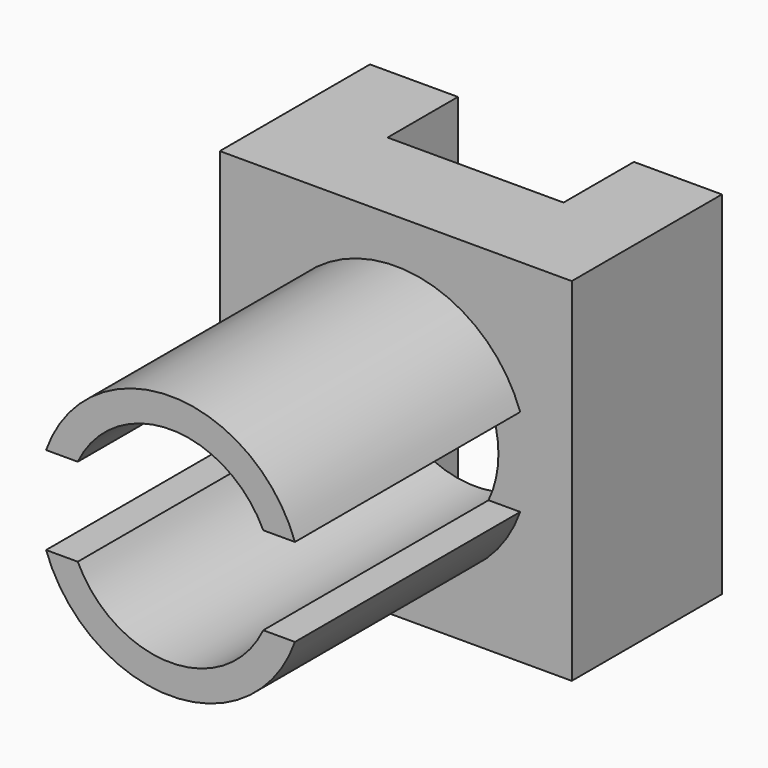
from build123d import *

# Parameters (mm, degrees)
F0_R     = 22.5
F0_R_2   = 17.5
F1_DEPTH = 48
F2_W     = 60
F2_H     = 60
F2_R     = 22.5
F2_R_2   = 17.5
F3_DEPTH = 32
F4_W     = 30
F4_H     = 15
F5_DEPTH = 60.001
F7_DEPTH = 48


with BuildPart() as f1:
    # F0 (on Front) → F1 (new body)
    with BuildSketch(Plane.XZ):
        Circle(F0_R)
        Circle(F0_R_2, mode=Mode.SUBTRACT)
    extrude(amount=F1_DEPTH)

    # F2 (on face) → F3 (join)
    with BuildSketch(Plane(origin=(0, 0, 0), x_dir=(-1, 0, 0), z_dir=(0, 1, 0))):
        Rectangle(F2_W, F2_H)
        Circle(F2_R, mode=Mode.SUBTRACT)
        Circle(F2_R)
        Circle(F2_R_2, mode=Mode.SUBTRACT)
    extrude(amount=F3_DEPTH)

    # F4 (on face) → F5 (cut, through all)
    with BuildSketch(Plane(origin=(0, 0, -30), x_dir=(1, 0, 0), z_dir=(0, 0, -1))):
        with Locations((0, -24.5)):
            Rectangle(F4_W, F4_H)
    extrude(amount=-F5_DEPTH, mode=Mode.SUBTRACT)

    # F6 (on face) → F7 (cut, through all)
    with BuildSketch(Plane.XZ.offset(48)):
        with BuildLine():
            ThreePointArc((-21.2132034356, 7.5), (-22.5, 0), (-21.2132034356, -7.5))
            Line((-21.2132034356, -7.5), (-15.8113883008, -7.5))
            ThreePointArc((-15.8113883008, -7.5), (-17.5, 0), (-15.8113883008, 7.5))
            Line((-15.8113883008, 7.5), (-21.2132034356, 7.5))
        make_face()
        with BuildLine():
            Line((15.8113883008, -7.5), (21.2132034356, -7.5))
            ThreePointArc((21.2132034356, -7.5), (22.1759675922, -3.8047945213), (22.5, 0))
            ThreePointArc((22.5, 0), (22.1759675922, 3.8047945213), (21.2132034356, 7.5))
            Line((21.2132034356, 7.5), (15.8113883008, 7.5))
            ThreePointArc((15.8113883008, 7.5), (17.0726286093, 3.843872054), (17.5, 0))
            ThreePointArc((17.5, 0), (17.0726286093, -3.843872054), (15.8113883008, -7.5))
        make_face()
    extrude(amount=-F7_DEPTH, mode=Mode.SUBTRACT)


solid = f1.part
